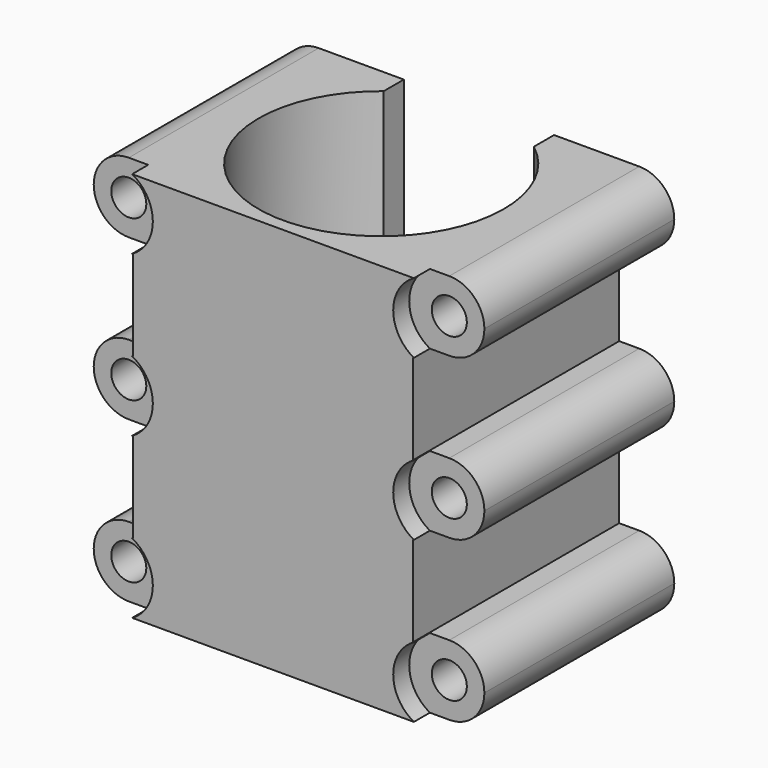
from build123d import *

# Parameters (mm, degrees)
F0_R           = 11.25
F1_DEPTH       = 39
F2_R           = 12.25
F2_R_2         = 11.25
F3_DEPTH       = 16
F5_R           = 0.99999
F4_R           = 12.25
F4_R_2         = 11.25
F6_DEPTH       = 10
F7_R           = 0.99999
F9_DEPTH       = 9
F11_DEPTH      = 39
F12_W          = 3.5
F12_H          = 5.5
F13_DEPTH      = 2
F13_DEPTH_BACK = 12
F15_DEPTH      = 2
F16_W          = 0.5
F16_H          = 4
F16_W_2        = 3
F17_DEPTH      = 6
F17_DEPTH_BACK = 16.7
F18_W          = 28
F18_H          = 39
F19_DEPTH      = 13.5
F19_DEPTH_BACK = 12.2
F21_R          = 1.75
F22_DEPTH      = 25.7
F24_R          = 1.75
F25_DEPTH      = 2


# Not quite as in the source:
# - a fillet or chamfer is up to 0.001 mm smaller than in the source, because OpenCascade refuses the exact size
# - a feature of the source that left no trace in its solid (it failed there, or was rolled back) is left out


with BuildPart() as f1:
    # F0 (on Top) → F1 (new body)
    with BuildSketch(Plane.XY):
        Circle(F0_R)
    extrude(amount=F1_DEPTH)

    # F2 (on face) → F3 (join)
    with BuildSketch(Plane.XY.offset(39)):
        Circle(F2_R)
        Circle(F2_R_2, mode=Mode.SUBTRACT)
    extrude(amount=-F3_DEPTH)

    # F5 (radius 1 in the source; OpenCascade refuses exactly that, so slightly less here)
    f5_edges = [f1.edges().sort_by_distance(p)[0] for p in [
        (-12.25, 0, 23),
    ]]
    fillet(f5_edges, radius=F5_R)

    # F4 (on face) → F6 (join)
    with BuildSketch(Plane(origin=(0, 0, 0), x_dir=(1, 0, 0), z_dir=(0, 0, -1))):
        Circle(F4_R)
        Circle(F4_R_2, mode=Mode.SUBTRACT)
    extrude(amount=-F6_DEPTH)

    # F7 (radius 1 in the source; OpenCascade refuses exactly that, so slightly less here)
    f7_edges = [f1.edges().sort_by_distance(p)[0] for p in [
        (-12.25, 0, 10),
    ]]
    fillet(f7_edges, radius=F7_R)

    # F8 (on face) → F9 (join)
    with BuildSketch(Plane(origin=(0, 0, 0), x_dir=(1, 0, 0), z_dir=(0, 0, -1))):
        with BuildLine():
            Line((0, 12.25), (-5.5, 12.25))
            Line((-5.5, 12.25), (-5.5, 10.9458896395))
            ThreePointArc((-5.5, 10.9458896395), (-2.8262476817, 11.9195144214), (0, 12.25))
        make_face()
        with BuildLine():
            Line((5.5, 12.25), (0, 12.25))
            ThreePointArc((0, 12.25), (2.8262476817, 11.9195144214), (5.5, 10.9458896395))
            Line((5.5, 10.9458896395), (5.5, 12.25))
        make_face()
    extrude(amount=-F9_DEPTH)

    # F10 (on face) → F11 (join)
    with BuildSketch(Plane(origin=(0, 0, 0), x_dir=(1, 0, 0), z_dir=(0, 0, -1))):
        with BuildLine():
            Line((7.5, -12.25), (7.5, -9.6856853139))
            ThreePointArc((7.5, -9.6856853139), (3.9631335396, -11.5912066907), (0, -12.25))
            Line((0, -12.25), (7.5, -12.25))
        make_face()
        with BuildLine():
            ThreePointArc((0, -12.25), (-3.9631335396, -11.5912066907), (-7.5, -9.6856853139))
            Line((-7.5, -9.6856853139), (-7.5, -12.25))
            Line((-7.5, -12.25), (0, -12.25))
        make_face()
        with BuildLine():
            Line((7.5, -8.25), (-7.5, -8.25))
            Line((-7.5, -8.25), (-7.5, -9.6856853139))
            ThreePointArc((-7.5, -9.6856853139), (-3.9631335396, -11.5912066907), (0, -12.25))
            ThreePointArc((0, -12.25), (3.9631335396, -11.5912066907), (7.5, -9.6856853139))
            Line((7.5, -9.6856853139), (7.5, -8.25))
        make_face()
    extrude(amount=-F11_DEPTH)

    # F12 (on face) → F13 (join, two sides)
    with BuildSketch(Plane(origin=(0, 12.25, 0), x_dir=(-1, 0, 0), z_dir=(0, 1, 0))) as f13_sk:
        with Locations((-9.25, 9.25)):
            Rectangle(F12_W, F12_H)
    extrude(amount=F13_DEPTH)
    extrude(f13_sk.sketch, amount=-F13_DEPTH_BACK)

    # F14 (on face) → F15 (join)
    with BuildSketch(Plane(origin=(0, 12.25, 0), x_dir=(-1, 0, 0), z_dir=(0, 1, 0))):
        with BuildLine():
            ThreePointArc((0, 25.4997491551), (-4.6734438866, 14.4240399421), (6.4428955234, 19))
            ThreePointArc((6.4428955234, 19), (4.5592349335, 23.5759600579), (0, 25.4997491551))
        make_face()
    extrude(amount=F15_DEPTH)

    # F16 (on face) → F17 (join, two sides)
    with BuildSketch(Plane(origin=(0, 12.25, 0), x_dir=(-1, 0, 0), z_dir=(0, 1, 0))) as f17_sk:
        with Locations((-7.75, 29.5)):
            Rectangle(F16_W, F16_H)
        with Locations((-6, 29.5)):
            Rectangle(F16_W_2, F16_H)
    extrude(amount=F17_DEPTH)
    extrude(f17_sk.sketch, amount=-F17_DEPTH_BACK)


with BuildPart() as f19:
    # F18 (on Front) → F19 (new body, two sides)
    with BuildSketch(Plane.XZ) as f19_sk:
        with Locations((0, 19.5)):
            Rectangle(F18_W, F18_H)
    extrude(amount=F19_DEPTH)
    extrude(f19_sk.sketch, amount=-F19_DEPTH_BACK)

    # F20: cut F1
    add(f1.part, mode=Mode.SUBTRACT)

    # F21 (on face) → F22 (join)
    with BuildSketch(Plane.XZ.offset(13.5)):
        with BuildLine():
            Line((-14, 0), (-14, 7))
            Line((-14, 7), (-16, 7))
            ThreePointArc((-16, 7), (-18.4748737342, 5.9748737342), (-19.5, 3.5))
            ThreePointArc((-19.5, 3.5), (-18.4748737342, 1.0251262658), (-16, 0))
            Line((-16, 0), (-14, 0))
        make_face()
        with Locations((-16, 3.5)):
            Circle(F21_R, mode=Mode.SUBTRACT)
        with BuildLine():
            Line((-16, 32), (-14, 32))
            Line((-14, 32), (-14, 39))
            Line((-14, 39), (-16, 39))
            ThreePointArc((-16, 39), (-18.4748737342, 37.9748737342), (-19.5, 35.5))
            ThreePointArc((-19.5, 35.5), (-18.4748737342, 33.0251262658), (-16, 32))
        make_face()
        with Locations((-16, 35.5)):
            Circle(F21_R, mode=Mode.SUBTRACT)
        with BuildLine():
            Line((14, 39), (14, 32))
            Line((14, 32), (16, 32))
            ThreePointArc((16, 32), (18.4748737342, 33.0251262658), (19.5, 35.5))
            ThreePointArc((19.5, 35.5), (18.4748737342, 37.9748737342), (16, 39))
            Line((16, 39), (14, 39))
        make_face()
        with Locations((16, 35.5)):
            Circle(F21_R, mode=Mode.SUBTRACT)
        with BuildLine():
            ThreePointArc((19.5, 3.5), (18.4748737342, 5.9748737342), (16, 7))
            Line((16, 7), (14, 7))
            Line((14, 7), (14, 0))
            Line((14, 0), (16, 0))
            ThreePointArc((16, 0), (18.4748737342, 1.0251262658), (19.5, 3.5))
        make_face()
        with Locations((16, 3.5)):
            Circle(F21_R, mode=Mode.SUBTRACT)
        with BuildLine():
            Line((-16, 16), (-14, 16))
            Line((-14, 16), (-14, 23))
            Line((-14, 23), (-16, 23))
            ThreePointArc((-16, 23), (-18.4748737342, 21.9748737342), (-19.5, 19.5))
            ThreePointArc((-19.5, 19.5), (-18.4748737342, 17.0251262658), (-16, 16))
        make_face()
        with Locations((-16, 19.5)):
            Circle(F21_R, mode=Mode.SUBTRACT)
        with BuildLine():
            Line((14, 23), (14, 16))
            Line((14, 16), (16, 16))
            ThreePointArc((16, 16), (18.4748737342, 17.0251262658), (19.5, 19.5))
            ThreePointArc((19.5, 19.5), (18.4748737342, 21.9748737342), (16, 23))
            Line((16, 23), (14, 23))
        make_face()
        with Locations((16, 19.5)):
            Circle(F21_R, mode=Mode.SUBTRACT)
    extrude(amount=-F22_DEPTH)

    # F24 (on face) → F25 (cut)
    with BuildSketch(Plane.XZ.offset(13.5)):
        with BuildLine():
            ThreePointArc((-14.0635083269, 32), (-12.5542804313, 33.4684939937), (-12, 35.5))
            ThreePointArc((-12, 35.5), (-12.5542804313, 37.5315060063), (-14.0635083269, 39))
            Line((-14.0635083269, 39), (-16, 39))
            ThreePointArc((-16, 39), (-19.5, 35.5), (-16, 32))
            Line((-16, 32), (-14.0635083269, 32))
        make_face()
        with Locations((-16, 35.5)):
            Circle(F24_R, mode=Mode.SUBTRACT)
        with BuildLine():
            Line((16, 39), (14.0635083269, 39))
            ThreePointArc((14.0635083269, 39), (12, 35.5), (14.0635083269, 32))
            Line((14.0635083269, 32), (16, 32))
            ThreePointArc((16, 32), (19.5, 35.5), (16, 39))
        make_face()
        with Locations((16, 35.5)):
            Circle(F24_R, mode=Mode.SUBTRACT)
        with BuildLine():
            Line((16, 7), (14.0635083269, 7))
            ThreePointArc((14.0635083269, 7), (12, 3.5), (14.0635083269, 0))
            Line((14.0635083269, 0), (16, 0))
            ThreePointArc((16, 0), (19.5, 3.5), (16, 7))
        make_face()
        with Locations((16, 3.5)):
            Circle(F24_R, mode=Mode.SUBTRACT)
        with BuildLine():
            ThreePointArc((-12, 3.5), (-12.5542804313, 5.5315060063), (-14.0635083269, 7))
            Line((-14.0635083269, 7), (-16, 7))
            ThreePointArc((-16, 7), (-19.5, 3.5), (-16, 0))
            Line((-16, 0), (-14.0635083269, 0))
            ThreePointArc((-14.0635083269, 0), (-12.5542804313, 1.4684939937), (-12, 3.5))
        make_face()
        with Locations((-16, 3.5)):
            Circle(F24_R, mode=Mode.SUBTRACT)
        with BuildLine():
            ThreePointArc((-12, 19.5), (-12.5542804313, 21.5315060063), (-14.0635083269, 23))
            Line((-14.0635083269, 23), (-16, 23))
            ThreePointArc((-16, 23), (-19.5, 19.5), (-16, 16))
            Line((-16, 16), (-14.0635083269, 16))
            ThreePointArc((-14.0635083269, 16), (-12.5542804313, 17.4684939937), (-12, 19.5))
        make_face()
        with Locations((-16, 19.5)):
            Circle(F24_R, mode=Mode.SUBTRACT)
        with BuildLine():
            Line((16, 23), (14.0635083269, 23))
            ThreePointArc((14.0635083269, 23), (12, 19.5), (14.0635083269, 16))
            Line((14.0635083269, 16), (16, 16))
            ThreePointArc((16, 16), (19.5, 19.5), (16, 23))
        make_face()
        with Locations((16, 19.5)):
            Circle(F24_R, mode=Mode.SUBTRACT)
    extrude(amount=-F25_DEPTH, mode=Mode.SUBTRACT)


solid = f19.part
